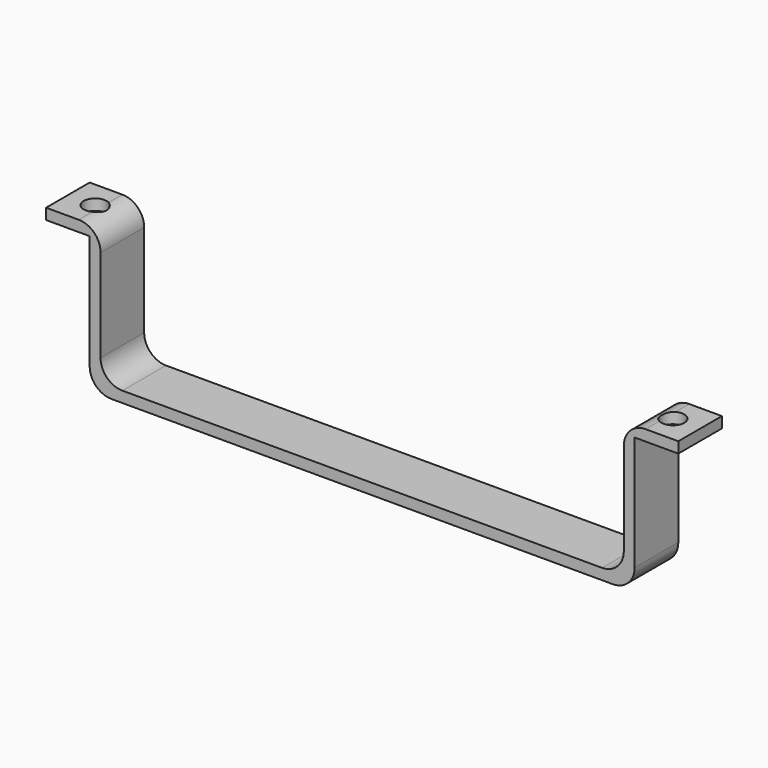
from build123d import *

# Parameters (mm, degrees)
F1_DEPTH    = 12.7
F2_R        = 2.667
F3_R        = 2.667
F4_DEPTH    = 25.4
F5_T1_DEPTH = 12.7
F5_T3_DEPTH = 38.1


# Not quite as in the source:
# - a fillet or chamfer that OpenCascade refuses, or shapes differently, is made with other operations: its cross-section is extruded or revolved along the edge and cut away or added


with BuildPart() as f1:
    # F0 (on Front) → F1 (new body)
    with BuildSketch(Plane.XZ):
        Polygon((121.92, 0), (0, 0), (0, 31.75), (-12.7, 31.75), (-12.7, 29.2099993676), (-2.5400006324, 29.2099993676), (-2.5400006324, -2.5400006324), (124.4600006324, -2.5400006324), (124.4600006324, 29.2099993676), (134.62, 29.2099993676), (134.62, 31.75), (121.92, 31.75), align=None)
    extrude(amount=F1_DEPTH)

    # F2 (on face) + F3 (on face) → F4 (cut)
    with BuildSketch(Plane.XY.offset(31.75)):
        with Locations((-6.35, -6.35)):
            Circle(F2_R)
    with BuildSketch(Plane.XY.offset(31.75)):
        with Locations((128.27, -6.35)):
            Circle(F3_R)
    extrude(amount=-F4_DEPTH, mode=Mode.SUBTRACT)

    # F5: fillet of radius 5.08 on 6 edges, made by hand

    # F5_s2 → F5_t1 (join)
    with BuildSketch(Plane.XZ):
        with BuildLine():
            ThreePointArc((5.08, 0), (1.4878975516, 1.4878975516), (0, 5.08))
            Line((0, 5.08), (0, 0))
            Line((0, 0), (5.08, 0))
        make_face()
        with BuildLine():
            ThreePointArc((116.84, 0), (120.4321024484, 1.4878975516), (121.92, 5.08))
            Line((121.92, 5.08), (121.92, 0))
            Line((121.92, 0), (116.84, 0))
        make_face()
    extrude(amount=F5_T1_DEPTH)

    # F5_s4 → F5_t3 (cut)
    with BuildSketch(Plane.XZ.offset(-12.7)):
        with BuildLine():
            ThreePointArc((-2.5400006324, 2.5399993676), (-1.0521030808, -1.0521030808), (2.5399993676, -2.5400006324))
            Line((2.5399993676, -2.5400006324), (-2.5400006324, -2.5400006324))
            Line((-2.5400006324, -2.5400006324), (-2.5400006324, 2.5399993676))
        make_face()
        with BuildLine():
            ThreePointArc((119.3800006324, -2.5400006324), (122.9721030808, -1.0521030808), (124.4600006324, 2.5399993676))
            Line((124.4600006324, 2.5399993676), (124.4600006324, -2.5400006324))
            Line((124.4600006324, -2.5400006324), (119.3800006324, -2.5400006324))
        make_face()
        with BuildLine():
            ThreePointArc((127, 31.75), (123.4078975516, 30.2621024484), (121.92, 26.67))
            Line((121.92, 26.67), (121.92, 31.75))
            Line((121.92, 31.75), (127, 31.75))
        make_face()
        with BuildLine():
            ThreePointArc((0, 26.67), (-1.4878975516, 30.2621024484), (-5.08, 31.75))
            Line((-5.08, 31.75), (0, 31.75))
            Line((0, 31.75), (0, 26.67))
        make_face()
    extrude(amount=F5_T3_DEPTH, mode=Mode.SUBTRACT)


solid = f1.part
